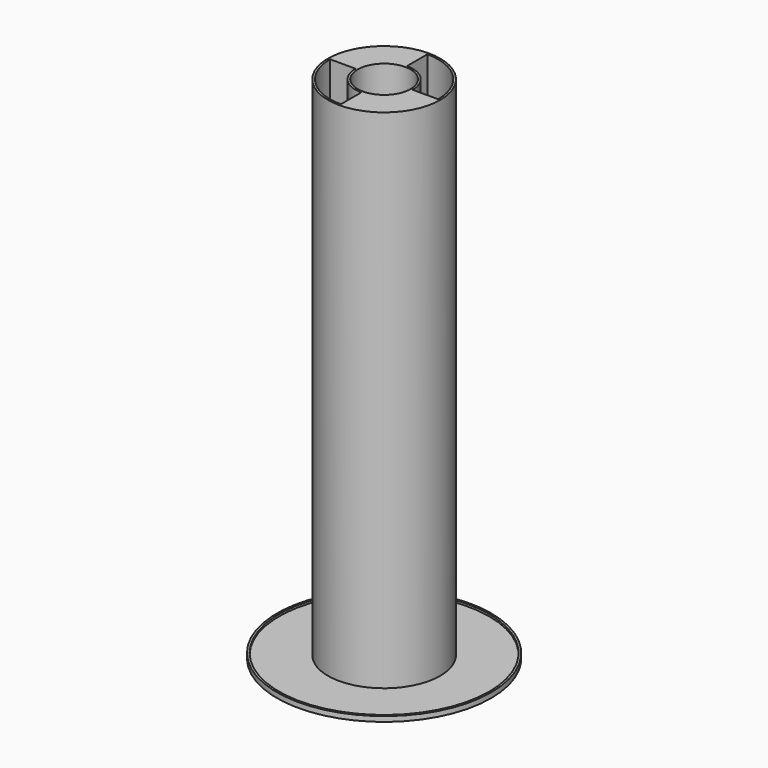
from build123d import *

# Parameters (mm, degrees)
F0_R     = 105
F0_R_2   = 55
F0_R_3   = 26
F1_DEPTH = 3
F2_DEPTH = 500
F3_DEPTH = 500
F4_R     = 105
F4_R_2   = 103
F5_DEPTH = 2
F6_DEPTH = 500
F7_DEPTH = 25


# Not quite as in the source:
# - after a boolean that leaves OpenCascade's solid faulty, fix() repairs it


with BuildPart() as f1:
    # F0 (on Top) → F1 (new body)
    with BuildSketch(Plane.XY):
        Circle(F0_R)
        Circle(F0_R_2, mode=Mode.SUBTRACT)
        Circle(F0_R_2)
        with BuildLine():
            ThreePointArc((0, 53), (37.4766594029, 37.4766594029), (53, 0))
            ThreePointArc((53, 0), (37.4766594029, -37.4766594029), (0, -53))
            ThreePointArc((0, -53), (-37.4766594029, -37.4766594029), (-53, 0))
            ThreePointArc((-53, 0), (-37.4766594029, 37.4766594029), (0, 53))
        make_face(mode=Mode.SUBTRACT)
        with BuildLine():
            ThreePointArc((0, 28), (19.7989898732, 19.7989898732), (28, 0))
            Line((28, 0), (53, 0))
            ThreePointArc((53, 0), (37.4766594029, 37.4766594029), (0, 53))
            Line((0, 53), (0, 28))
        make_face()
        with BuildLine():
            ThreePointArc((-28, 0), (-19.7989898732, 19.7989898732), (0, 28))
            Line((0, 28), (0, 53))
            ThreePointArc((0, 53), (-37.4766594029, 37.4766594029), (-53, 0))
            Line((-53, 0), (-28, 0))
        make_face()
        with BuildLine():
            Line((0, -53), (0, -28))
            ThreePointArc((0, -28), (-19.7989898732, -19.7989898732), (-28, 0))
            Line((-28, 0), (-53, 0))
            ThreePointArc((-53, 0), (-37.4766594029, -37.4766594029), (0, -53))
        make_face()
        with BuildLine():
            Line((53, 0), (28, 0))
            ThreePointArc((28, 0), (19.7989898732, -19.7989898732), (0, -28))
            Line((0, -28), (0, -53))
            ThreePointArc((0, -53), (37.4766594029, -37.4766594029), (53, 0))
        make_face()
        with BuildLine():
            ThreePointArc((0, -28), (19.7989898732, -19.7989898732), (28, 0))
            ThreePointArc((28, 0), (19.7989898732, 19.7989898732), (0, 28))
            ThreePointArc((0, 28), (-19.7989898732, 19.7989898732), (-28, 0))
            ThreePointArc((-28, 0), (-19.7989898732, -19.7989898732), (0, -28))
        make_face()
        Circle(F0_R_3, mode=Mode.SUBTRACT)
    extrude(amount=F1_DEPTH)

    # F0 (on Top) → F2 (join)
    with BuildSketch(Plane.XY):
        with BuildLine():
            ThreePointArc((0, -28), (19.7989898732, -19.7989898732), (28, 0))
            ThreePointArc((28, 0), (19.7989898732, 19.7989898732), (0, 28))
            ThreePointArc((0, 28), (-19.7989898732, 19.7989898732), (-28, 0))
            ThreePointArc((-28, 0), (-19.7989898732, -19.7989898732), (0, -28))
        make_face()
        Circle(F0_R_3, mode=Mode.SUBTRACT)
    extrude(amount=F2_DEPTH)

    # F0 (on Top) → F3 (join)
    with BuildSketch(Plane.XY):
        Circle(F0_R_2)
        with BuildLine():
            ThreePointArc((0, 53), (37.4766594029, 37.4766594029), (53, 0))
            ThreePointArc((53, 0), (37.4766594029, -37.4766594029), (0, -53))
            ThreePointArc((0, -53), (-37.4766594029, -37.4766594029), (-53, 0))
            ThreePointArc((-53, 0), (-37.4766594029, 37.4766594029), (0, 53))
        make_face(mode=Mode.SUBTRACT)
    extrude(amount=F3_DEPTH)

    # F4 (on face) → F5 (join)
    with BuildSketch(Plane.XY.offset(3)):
        Circle(F4_R)
        Circle(F4_R_2, mode=Mode.SUBTRACT)
    extrude(amount=F5_DEPTH)

    # F0 (on Top) → F6 (join)
    with BuildSketch(Plane.XY):
        with BuildLine():
            ThreePointArc((-28, 0), (-19.7989898732, 19.7989898732), (0, 28))
            Line((0, 28), (0, 53))
            ThreePointArc((0, 53), (-37.4766594029, 37.4766594029), (-53, 0))
            Line((-53, 0), (-28, 0))
        make_face()
        with BuildLine():
            Line((53, 0), (28, 0))
            ThreePointArc((28, 0), (19.7989898732, -19.7989898732), (0, -28))
            Line((0, -28), (0, -53))
            ThreePointArc((0, -53), (37.4766594029, -37.4766594029), (53, 0))
        make_face()
    extrude(amount=F6_DEPTH)

    # F0 (on Top) → F7 (cut)
    with BuildSketch(Plane.XY):
        with BuildLine():
            Line((0, -53), (0, -28))
            ThreePointArc((0, -28), (-19.7989898732, -19.7989898732), (-28, 0))
            Line((-28, 0), (-53, 0))
            ThreePointArc((-53, 0), (-37.4766594029, -37.4766594029), (0, -53))
        make_face()
        with BuildLine():
            ThreePointArc((0, 28), (19.7989898732, 19.7989898732), (28, 0))
            Line((28, 0), (53, 0))
            ThreePointArc((53, 0), (37.4766594029, 37.4766594029), (0, 53))
            Line((0, 53), (0, 28))
        make_face()
    extrude(amount=F7_DEPTH, mode=Mode.SUBTRACT)

    add(f1.part.fix(), mode=Mode.REPLACE)


solid = f1.part
